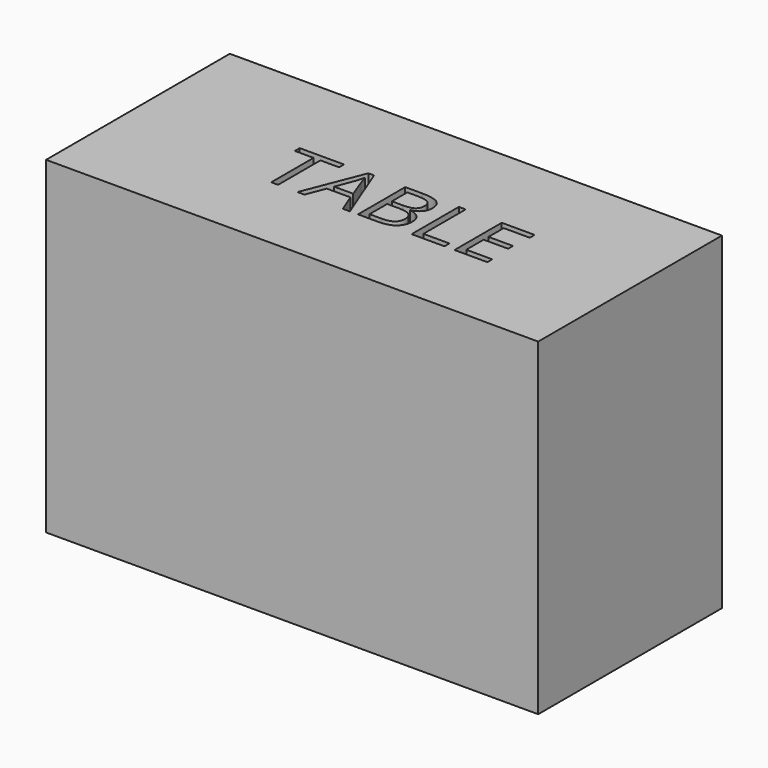
from build123d import *

# Parameters (mm, degrees)
F0_W         = 1500
F0_H         = 700
F1_DEPTH     = 1000
F2_TEXT_SIZE = 252.0895666546
F3_DEPTH     = 111


# Not quite as in the source:
# - Text() gives the source's letters only with a copy of the font that has no kerning and outlines rounded to 1/6400 em; it was checked with that copy


with BuildPart() as f1:
    # F0 (on Top) → F1 (new body)
    with BuildSketch(Plane.XY):
        with Locations((730.9079031476, 343.5845352566)):
            Rectangle(F0_W, F0_H)
    extrude(amount=F1_DEPTH)

    # F2 (on face) → F3 (cut)
    with BuildSketch(Plane.XY.offset(1000)):
        with Locations((412.5578403473, 237.7225756645)):
            Text('TABLE', F2_TEXT_SIZE, font='Open Sans', text_align=(TextAlign.LEFT, TextAlign.BOTTOM))
    extrude(amount=-F3_DEPTH, mode=Mode.SUBTRACT)


solid = f1.part
